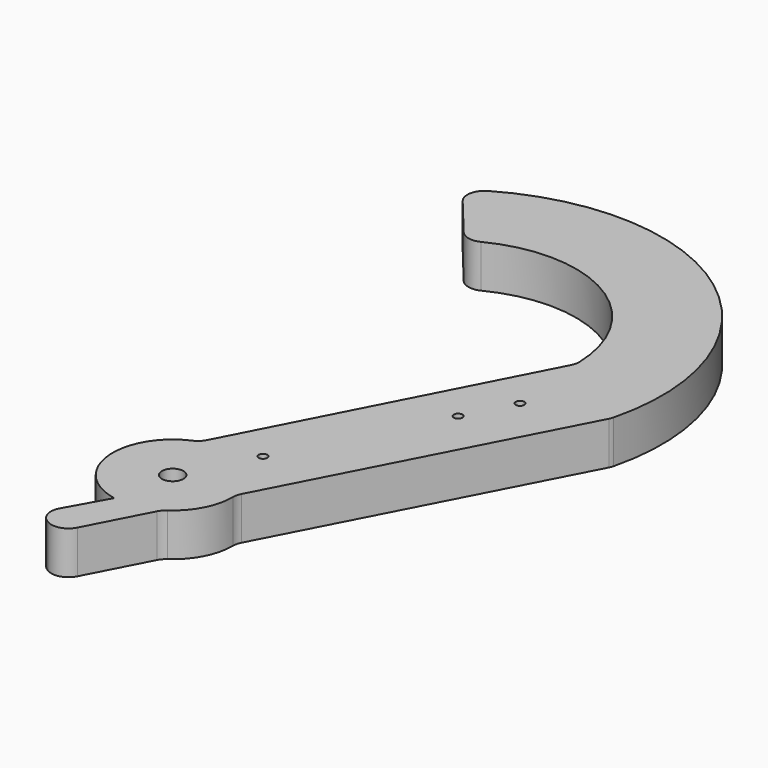
from build123d import *

# Parameters (mm, degrees)
F0_R     = 1.25
F0_R_2   = 0.5
F1_DEPTH = 5
F2_R     = 2


# Not quite as in the source:
# - two fillets or chamfers of one size are made in one step
# - a feature names something its author has since deleted; it is built from what else it names


with BuildPart() as f1:
    # F0 (on Top) → F1 (new body)
    with BuildSketch(Plane.XY):
        with BuildLine():
            Line((-14.5326076762, 20.3421560836), (-8.1431852604, 12.5971637211))
            ThreePointArc((-8.1431852604, 12.5971637211), (7.1712000772, 13.174744379), (15, 0))
            Line((15, 0), (-2.1995428838, -33.3545495937))
            ThreePointArc((-2.1995428838, -33.3545495937), (-6.9846930225, -40.4626698406), (-1.3037745428, -46.8775120459))
            ThreePointArc((-1.3037745428, -46.8775120459), (1.2316251761, -46.8907981704), (3.6054450158, -46.0000638528))
            Line((3.6054450158, -46.0000638528), (6.9816735201, -39.4938035379))
            Line((6.9816735201, -39.4938035379), (24.1795416276, -6.3521466198))
            ThreePointArc((24.1795416276, -6.3521466198), (14.1919795262, 20.5812467341), (-14.5326076762, 20.3421560836))
        make_face()
        with Locations((0, -40)):
            Circle(F0_R, mode=Mode.SUBTRACT)
        with Locations((4.1248112098, -32.0008792681)):
            Circle(F0_R_2, mode=Mode.SUBTRACT)
        with Locations((13.0337394799, -14.7240660517)):
            Circle(F0_R_2, mode=Mode.SUBTRACT)
        with Locations((15.8593580654, -9.2444300009)):
            Circle(F0_R_2, mode=Mode.SUBTRACT)
        with BuildLine():
            ThreePointArc((3.6054450158, -46.0000638528), (1.2316251761, -46.8907981704), (-1.3037745428, -46.8775120459))
            Line((-1.3037745428, -46.8775120459), (-4.8843406974, -53.3048406851))
            Line((-4.8843406974, -53.3048406851), (-1.2389638203, -55.3356242034))
            Line((-1.2389638203, -55.3356242034), (3.6054450158, -46.0000638528))
        make_face()
        with BuildLine():
            ThreePointArc((3.6054450158, -46.0000638528), (6.2132620695, -43.2241858593), (6.9816735201, -39.4938035379))
            Line((6.9816735201, -39.4938035379), (3.6054450158, -46.0000638528))
        make_face()
    extrude(amount=F1_DEPTH)

    # F2
    f2_edges = [f1.edges().sort_by_distance(p)[0] for p in [
        (6.981674, -39.493804, 2.5),
        (15, 0, 2.5),
        (-8.143185, 12.597164, 2.5),
        (-14.532608, 20.342156, 2.5),
        (24.179542, -6.352147, 2.5),
        (-2.199543, -33.35455, 2.5),
        (-4.884341, -53.304841, 2.5),
        (-1.238964, -55.335624, 2.5),
        (3.605445, -46.000064, 2.5),
    ]]
    fillet(f2_edges, radius=F2_R)


solid = f1.part
